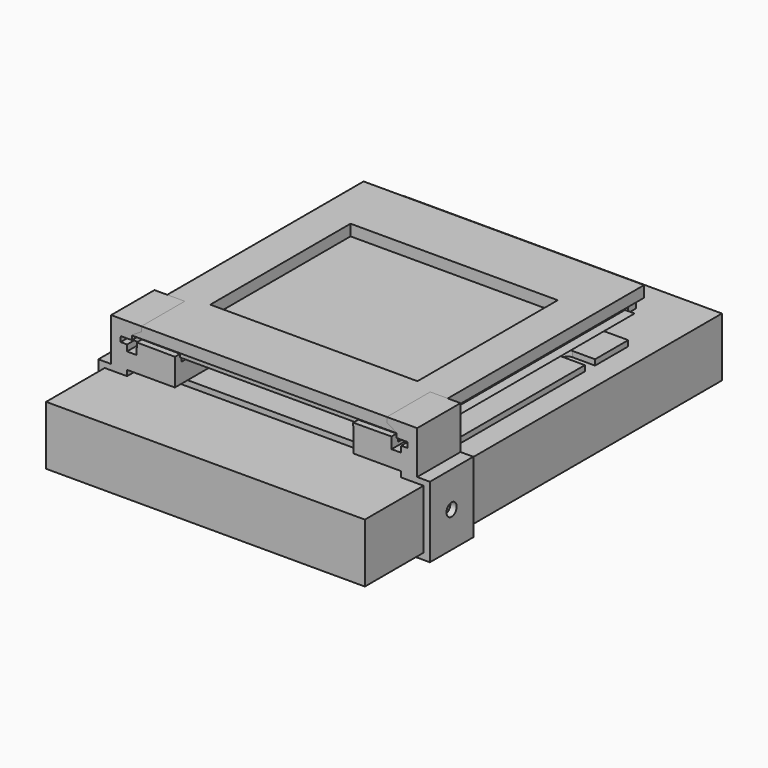
from build123d import *

# Parameters (mm, degrees)
F0_W           = 100
F0_H           = 140
F1_DEPTH       = 18.5
F3_DEPTH       = 1.75
F4_W           = 65
F4_H           = 55
F5_DEPTH       = 10
F6_W           = 88
F6_H           = 94
F6_W_2         = 86
F6_H_2         = 84
F6_W_3         = 65
F6_H_3         = 55
F6_H_4         = 3
F7_DEPTH       = 3.5
F8_DEPTH       = 2.5
F9_W           = 1
F9_H           = 1.25
F10_DEPTH      = 42
F10_DEPTH_BACK = 42
F12_DEPTH      = 47
F13_DEPTH      = 30
F15_DEPTH      = 12
F17_DEPTH      = 17
F19_DEPTH      = 40
F20_R          = 2
F21_DEPTH      = 120


with BuildPart() as f1:
    # F0 (on Top) → F1 (new body)
    with BuildSketch(Plane.XY):
        Rectangle(F0_W, F0_H)
    extrude(amount=-F1_DEPTH)


with BuildPart() as f3:
    # F2 (on Top) → F3 (new body)
    with BuildSketch(Plane.XY):
        with BuildLine():
            Line((43, 42), (-43, 42))
            Line((-43, 42), (-43, 29))
            Line((-43, 29), (-36, 29))
            ThreePointArc((-36, 29), (-34, 27), (-36, 25))
            Line((-36, 25), (-43, 25))
            Line((-43, 25), (-43, -25))
            Line((-43, -25), (-36, -25))
            ThreePointArc((-36, -25), (-34, -27), (-36, -29))
            Line((-36, -29), (-43, -29))
            Line((-43, -29), (-43, -42))
            Line((-43, -42), (43, -42))
            Line((43, -42), (43, -29))
            Line((43, -29), (36, -29))
            ThreePointArc((36, -29), (34, -27), (36, -25))
            Line((36, -25), (43, -25))
            Line((43, -25), (43, 25))
            Line((43, 25), (36, 25))
            ThreePointArc((36, 25), (34, 27), (36, 29))
            Line((36, 29), (43, 29))
            Line((43, 29), (43, 42))
        make_face()
    extrude(amount=F3_DEPTH)


with BuildPart() as f5:
    # F4 (on face) → F5 (new body)
    with BuildSketch(Plane.XY.offset(1.75)):
        Rectangle(F4_W, F4_H)
    extrude(amount=F5_DEPTH)


with BuildPart() as f7:
    # F6 (on face) → F7 (new body)
    with BuildSketch(Plane.XY.offset(11.75)):
        Rectangle(F6_W, F6_H)
        Polygon((-43, 42), (-43, 45), (43, 45), (43, 42), (43, -42), (43, -44), (43, -45), (-43, -45), (-43, -44), (-43, -42), align=None, mode=Mode.SUBTRACT)
        Rectangle(F6_W_2, F6_H_2)
        Rectangle(F6_W_3, F6_H_3, mode=Mode.SUBTRACT)
        with Locations((0, 43.5)):
            Rectangle(F6_W_2, F6_H_4)
        Polygon((43, -42), (-43, -42), (-43, -44), (-43, -45), (43, -45), (43, -44), align=None)
    extrude(amount=F7_DEPTH)

    # F6 (on face) → F8 (join)
    with BuildSketch(Plane.XY.offset(11.75)):
        with Locations((0, 43.5)):
            Rectangle(F6_W_2, F6_H_4)
        Polygon((43, -42), (-43, -42), (-43, -44), (-43, -45), (43, -45), (43, -44), align=None)
    extrude(amount=-F8_DEPTH)

    # F9 (on Front) → F10 (join, two sides)
    with BuildSketch(Plane.XZ) as f10_sk:
        with Locations((42.5, 9.125)):
            Rectangle(F9_W, F9_H)
        Polygon((43, 9.75), (43, 8.5), (45, 9.75), align=None)
    extrude(amount=F10_DEPTH)
    extrude(f10_sk.sketch, amount=-F10_DEPTH_BACK)


with BuildPart() as f12:
    # F11 (on Front) → F12 (new body)
    with BuildSketch(Plane.XZ):
        Polygon((27.9699712028, 6.7499098263), (28, 1.75), (43, 1.75), (43, 0), (48, 0), (50, 0), (52, 0), (52, 1.75), (48, 1.75), (48, 13.75), (48, 15.25), (38.5, 15.25), (38.5, 13.75), (41.5, 11.875), (41.5, 10.4472711682), (44.9731051922, 10.4472711682), (45, 8.7854899466), (43, 8.7531212961), (43, 6.8401781918), align=None)
        Polygon((52, 0), (50, 0), (50, -18.5), (35.7036739588, -18.5), (35.7036739588, -20.5), (52, -20.5), align=None)
    extrude(amount=F12_DEPTH)

    # F11 (on Front) → F13 (cut)
    with BuildSketch(Plane.XZ):
        Polygon((27.9699712028, 6.7499098263), (28, 1.75), (43, 1.75), (43, 0), (48, 0), (50, 0), (52, 0), (52, 1.75), (48, 1.75), (48, 13.75), (48, 15.25), (38.5, 15.25), (38.5, 13.75), (41.5, 11.875), (41.5, 10.4472711682), (44.9731051922, 10.4472711682), (45, 8.7854899466), (43, 8.7531212961), (43, 6.8401781918), align=None)
        Polygon((52, 0), (50, 0), (50, -18.5), (35.7036739588, -18.5), (35.7036739588, -20.5), (52, -20.5), align=None)
    extrude(amount=F13_DEPTH, mode=Mode.SUBTRACT)

    # F14 (on face) → F15 (join)
    with BuildSketch(Plane(origin=(28.0094999534, 0, 0.1682213529), x_dir=(0, -1, 0), z_dir=(-0.9999819653, 0, -0.0060057594))):
        Polygon((39.5, 5.9370710514), (47, 5.9370710514), (47, 7.0816674463), (47, 10.0810629427), (44.5, 10.0810629427), (44.5, 7.5816674463), (42, 7.5816674463), (42, 9.5810629427), (42, 10.0810629427), (39.5, 10.0810629427), (39.5, 9.5810629427), align=None)
    extrude(amount=-F15_DEPTH)


with BuildPart() as f17:
    # F16 (on face) → F17 (new body)
    with BuildSketch(Plane.XZ.offset(47)):
        Polygon((-35.7036739588, -20.5), (-35.7036739588, -18.5), (-50, -18.5), (-50, 0), (-43, 0), (-43, 1.75), (-28, 1.75), (-27.9489555144, 10.2491024863), (-39.9487390975, 10.3211715997), (-39.9697547859, 6.8219789397), (-43, 6.8401781918), (-43, 8.7531212961), (-45, 8.7854899466), (-44.9731051922, 10.4472711682), (-41.5, 10.4472711682), (-41.5, 11.875), (-38.5, 13.75), (-38.5, 15.25), (-48, 15.25), (-48, 1.75), (-52, 1.75), (-52, -20.5), align=None)
    extrude(amount=-F17_DEPTH)

    # F18 (on Right) → F19 (cut)
    with BuildSketch(Plane.YZ):
        Polygon((-39.5, 10.4472711682), (-39.5, 10.2491024863), (-39.5, 6.8401781918), (-30, 6.8401781918), (-30, 10.2491024863), (-30, 10.4472711682), align=None)
        Polygon((-44.5, 10.4472711682), (-44.5, 10.2491024863), (-44.5, 7.8218211792), (-42, 7.8218211792), (-42, 10.2491024863), (-42, 10.4472711682), align=None)
    extrude(amount=-F19_DEPTH, mode=Mode.SUBTRACT)


with BuildPart() as f21_tool:
    # F20 (on face) → F21 (new body)
    with BuildSketch(Plane.YZ.offset(52)):
        with Locations((-38.5, -9.375)):
            Circle(F20_R)
    extrude(amount=-F21_DEPTH)


with BuildPart() as f12_1:
    add(f12.part)

    # F21: cut by f21_tool
    add(f21_tool.part, mode=Mode.SUBTRACT)


with BuildPart() as f17_1:
    add(f17.part)

    # F21: cut by f21_tool
    add(f21_tool.part, mode=Mode.SUBTRACT)


solid = Compound([f1.part, f3.part, f5.part, f7.part, f12_1.part, f17_1.part])
